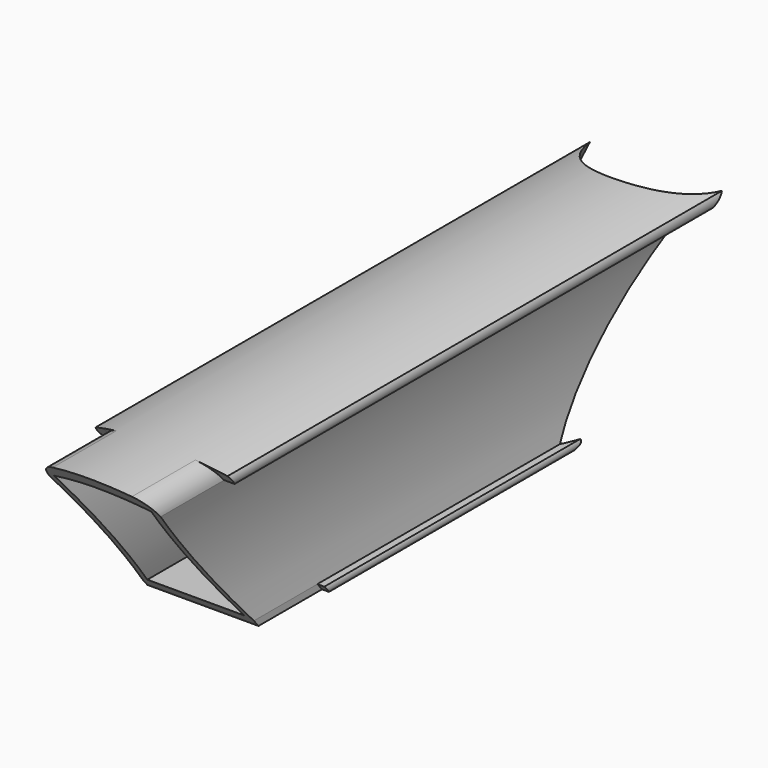
from build123d import *

# Parameters (mm, degrees)
F1_DEPTH       = 207.9847365
F2_T1_DEPTH    = 312.4469684912
F3_T1_DEPTH    = 284.4287008275
F6_START       = -2
F6_DEPTH       = 4
F9_START       = 2
F9_DEPTH       = 4
F11_R          = 20
F12_DEPTH      = 90
F12_DEPTH_BACK = 5
F13_T4_DEPTH   = 46.8692709023
F13_T9_DEPTH   = 46.8692709023


# Not quite as in the source:
# - a fillet or chamfer that OpenCascade refuses, or shapes differently, is made with other operations: its cross-section is extruded or revolved along the edge and cut away or added


with BuildPart() as f1:
    # F0 (on Front) → F1 (new body)
    with BuildSketch(Plane.XZ):
        with BuildLine():
            Line((-18, 0), (0, 0))
            Line((0, 0), (18, 0))
            ThreePointArc((18, 0), (18.2679491924, 1), (18, 2))
            Line((18, 2), (16, 2))
            ThreePointArc((16, 2), (13.9795897113, 22), (16, 42))
            Line((16, 42), (19, 42))
            ThreePointArc((19, 42), (19.4019237886, 43.5), (19, 45))
            ThreePointArc((19, 45), (0, 48.7506756806), (-19, 45))
            ThreePointArc((-19, 45), (-19.4019237886, 43.5), (-19, 42))
            Line((-19, 42), (-16, 42))
            ThreePointArc((-16, 42), (-13.9795897113, 22), (-16, 2))
            Line((-16, 2), (-18, 2))
            ThreePointArc((-18, 2), (-18.2679491924, 1), (-18, 0))
        make_face()
        with BuildLine():
            Line((14, 3), (0, 3))
            Line((0, 3), (-14, 3))
            ThreePointArc((-14, 3), (-11.9795897113, 23), (-14, 43))
            ThreePointArc((-14, 43), (0, 45), (14, 43))
            ThreePointArc((14, 43), (11.9795897113, 23), (14, 3))
        make_face(mode=Mode.SUBTRACT)
    extrude(amount=F1_DEPTH)

    # F2: chamfer of 45 x 53.6289116667 on 1 edges, made by hand

    # F2_s2 → F2_t1 (cut)
    with BuildSketch(Plane.YZ.offset(-156.2234842456)):
        Polygon((-207.9847365, 53.6289116667), (-162.9847365, 0), (-207.9847365, 0), align=None)
    extrude(amount=F2_T1_DEPTH, mode=Mode.SUBTRACT)

    # F3: chamfer of 45 x 48.2565919511 on 1 edges, made by hand

    # F3_s2 → F3_t1 (cut)
    with BuildSketch(Plane.YZ.offset(-142.2143504137)):
        Polygon((0, 45), (-48.2565919511, 0), (0, 0), align=None)
    extrude(amount=F3_T1_DEPTH, mode=Mode.SUBTRACT)

    # F5 (on face) → F6 (cut)
    with BuildSketch(Plane(origin=(14, 0, 0), x_dir=(0, -1, 0), z_dir=(-1, 0, 0)).offset(F6_START)):
        Polygon((200.7156460232, 72.1911139462), (140.1401089367, 0), (198.049341578, 0), (232.2688040982, 72.1911139462), align=None)
    extrude(amount=-F6_DEPTH, mode=Mode.SUBTRACT)

    # F8 (on face) → F9 (cut)
    with BuildSketch(Plane(origin=(-14, 0, 0), x_dir=(0, -1, 0), z_dir=(-1, 0, 0)).offset(F9_START)):
        Polygon((185.9322765967, 54.5729803215), (140.1401089367, 0), (168.9397689519, 0), (210.618345394, 54.5729803215), align=None)
    extrude(amount=F9_DEPTH, mode=Mode.SUBTRACT)

    # F11 (on face) → F12 (cut, two sides)
    with BuildSketch(Plane(origin=(0, 22.4451911308, 20.9304793408), x_dir=(-1, 0, 0), z_dir=(0, 0.7313537016, 0.6819983601))) as f12_sk:
        with Locations((0, 26.6659185749)):
            Circle(F11_R)
    extrude(amount=-F12_DEPTH, mode=Mode.SUBTRACT)
    extrude(f12_sk.sketch, amount=F12_DEPTH_BACK, mode=Mode.SUBTRACT)

    # F13: fillet of radius 6 on 2 edges, made by hand


with BuildPart() as f13_tool2:
    # F13_s3 → F13_t4 (new body)
    with BuildSketch(Plane.XZ.offset(213.6976361216)):
        with BuildLine():
            ThreePointArc((11.3791048339, 47.4386205251), (14.5860497205, 45.4810144553), (16, 42))
            Line((16, 42), (16, 46.1215528099))
            ThreePointArc((16, 46.1215528099), (13.7053826002, 46.8356264218), (11.3791048339, 47.4386205251))
        make_face()
    extrude(amount=-F13_T4_DEPTH)

    split(bisect_by=Plane(origin=(0, -82.2375917358, -69.0055328944), x_dir=(1, 0, 0), z_dir=(0, -0.7660444431, -0.6427876097)), keep=Keep.TOP)


with BuildPart() as f1_1:
    add(f1.part)

    # F13_t1: cut F13_tool2
    add(f13_tool2.part, mode=Mode.SUBTRACT)


with BuildPart() as f13_tool7:
    # F13_s8 → F13_t9 (new body)
    with BuildSketch(Plane.XZ.offset(213.6976361216)):
        with BuildLine():
            ThreePointArc((-16, 42), (-14.5860497205, 45.4810144553), (-11.3791048339, 47.4386205251))
            ThreePointArc((-11.3791048339, 47.4386205251), (-13.7053826002, 46.8356264218), (-16, 46.1215528099))
            Line((-16, 46.1215528099), (-16, 42))
        make_face()
    extrude(amount=-F13_T9_DEPTH)

    split(bisect_by=Plane(origin=(0, -82.2375917358, -69.0055328944), x_dir=(1, 0, 0), z_dir=(0, -0.7660444431, -0.6427876097)), keep=Keep.TOP)


with BuildPart() as f1_2:
    add(f1_1.part)

    # F13_t6: cut F13_tool7
    add(f13_tool7.part, mode=Mode.SUBTRACT)


solid = f1_2.part
